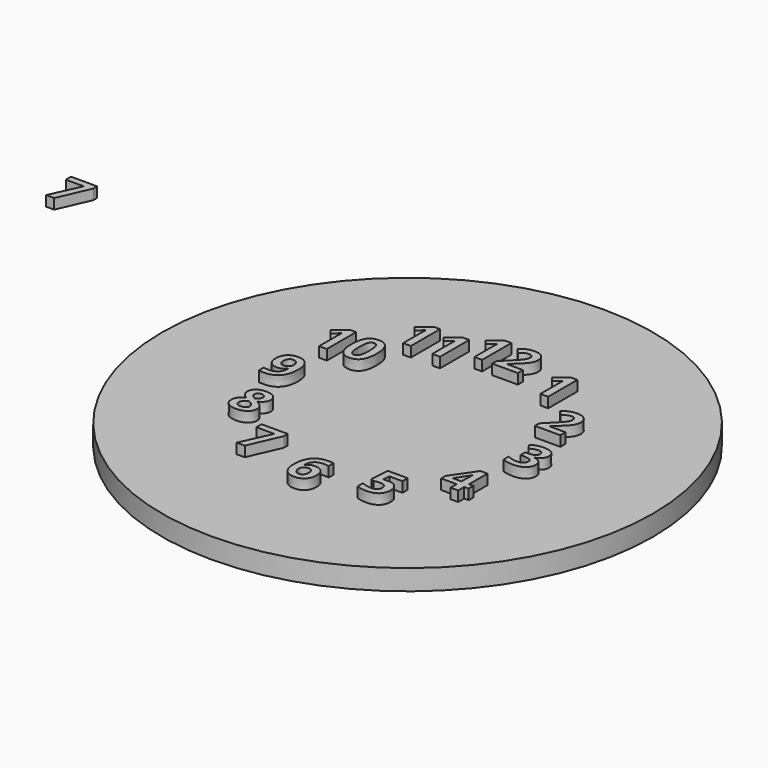
from build123d import *

# Parameters (mm, degrees)
F0_R         = 76.2
F1_DEPTH     = 6.35
F2_TEXT_SIZE = 15.875
F3_DEPTH     = 3.175


# Not quite as in the source:
# - Text() gives the source's letters only with a copy of the font that has no kerning and outlines rounded to 1/6400 em; it was checked with that copy


with BuildPart() as f1:
    # F0 (on Top) → F1 (new body)
    with BuildSketch(Plane.XY):
        Circle(F0_R)
    extrude(amount=-F1_DEPTH)


with BuildPart() as f3:
    # F2 (on Top) → F3 (new body)
    with BuildSketch(Plane.XY):
        with Locations((15.2561230469, 27.2805678842)):
            Text('1', F2_TEXT_SIZE, font='Open Sans', font_style=FontStyle.BOLD, text_align=(TextAlign.LEFT, TextAlign.BOTTOM))
        with Locations((28.2020620248, 13.335)):
            Text('2', F2_TEXT_SIZE, font='Open Sans', font_style=FontStyle.BOLD, text_align=(TextAlign.LEFT, TextAlign.BOTTOM))
        with Locations((33.3610644531, -5.715)):
            Text('3', F2_TEXT_SIZE, font='Open Sans', font_style=FontStyle.BOLD, text_align=(TextAlign.LEFT, TextAlign.BOTTOM))
        with Locations((28.0743178842, -24.765)):
            Text('4', F2_TEXT_SIZE, font='Open Sans', font_style=FontStyle.BOLD, text_align=(TextAlign.LEFT, TextAlign.BOTTOM))
        with Locations((14.3606738281, -38.7105678842)):
            Text('5', F2_TEXT_SIZE, font='Open Sans', font_style=FontStyle.BOLD, text_align=(TextAlign.LEFT, TextAlign.BOTTOM))
        with Locations((-4.7935058594, -43.815)):
            Text('6', F2_TEXT_SIZE, font='Open Sans', font_style=FontStyle.BOLD, text_align=(TextAlign.LEFT, TextAlign.BOTTOM))
        with Locations((-23.8435058594, -38.7105678842)):
            Text('7', F2_TEXT_SIZE, font='Open Sans', font_style=FontStyle.BOLD, text_align=(TextAlign.LEFT, TextAlign.BOTTOM))
        with Locations((-37.7655092904, -24.765)):
            Text('8', F2_TEXT_SIZE, font='Open Sans', font_style=FontStyle.BOLD, text_align=(TextAlign.LEFT, TextAlign.BOTTOM))
        with Locations((-42.8699414063, -5.715)):
            Text('9', F2_TEXT_SIZE, font='Open Sans', font_style=FontStyle.BOLD, text_align=(TextAlign.LEFT, TextAlign.BOTTOM))
        with Locations((-42.2886440561, 13.335)):
            Text('10', F2_TEXT_SIZE, font='Open Sans', font_style=FontStyle.BOLD, text_align=(TextAlign.LEFT, TextAlign.BOTTOM))
        with Locations((-27.374453125, 27.2805678842)):
            Text('11', F2_TEXT_SIZE, font='Open Sans', font_style=FontStyle.BOLD, text_align=(TextAlign.LEFT, TextAlign.BOTTOM))
        with Locations((-9.3240820313, 32.385)):
            Text('12', F2_TEXT_SIZE, font='Open Sans', font_style=FontStyle.BOLD, text_align=(TextAlign.LEFT, TextAlign.BOTTOM))
        with Locations((-141.0969942808, 33.90899948)):
            Text('7', F2_TEXT_SIZE, font='Open Sans', font_style=FontStyle.BOLD, text_align=(TextAlign.LEFT, TextAlign.BOTTOM))
    extrude(amount=F3_DEPTH)


solid = Compound([f1.part, f3.part])
